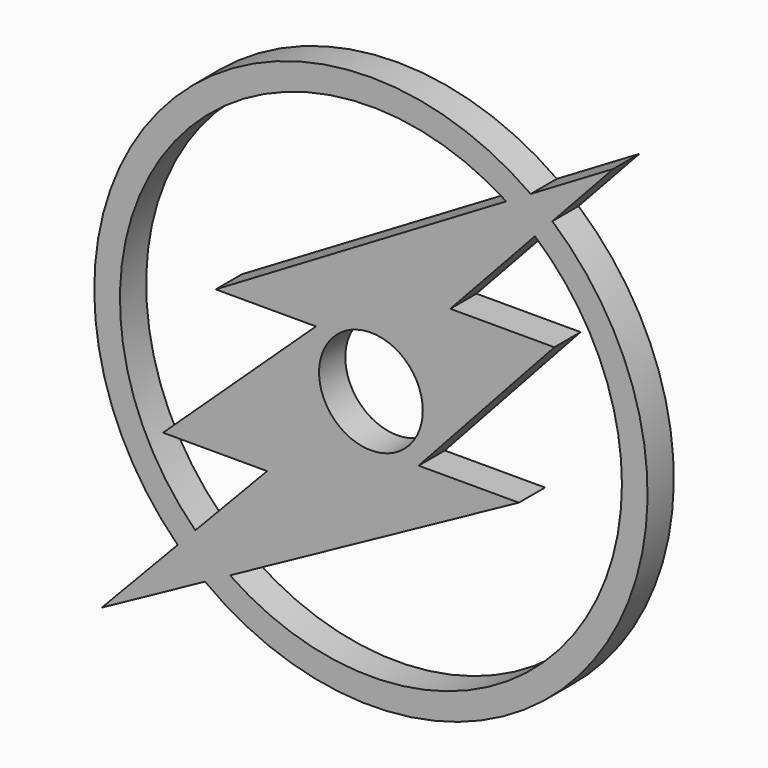
from build123d import *

# Parameters (mm, degrees)
F0_R     = 10.9728
F1_DEPTH = 6.9342


# Not quite as in the source:
# - a feature names something its author has since deleted; it is built from what else it names


with BuildPart() as f1:
    # F0 (on Front) → F1 (new body)
    with BuildSketch(Plane.XZ):
        with BuildLine():
            ThreePointArc((28.6439371533, 44.738406593), (31.7550616118, 42.5865732614), (34.7051660635, 40.2187967078))
            Line((34.7051660635, 40.2187967078), (38.3958422982, 44.2064153225))
            ThreePointArc((38.3958422982, 44.2064153225), (36.1509937048, 46.060324745), (33.8167671779, 47.8003568929))
            Line((33.8167671779, 47.8003568929), (28.6439371533, 44.738406593))
        make_face()
        with BuildLine():
            Line((38.3958422982, 44.2064153225), (34.7051660635, 40.2187967078))
            ThreePointArc((34.7051660635, 40.2187967078), (48.2991997583, 22.1175826623), (53.1225014483, 0))
            ThreePointArc((53.1225014483, 0), (24.8760182095, -46.9380855826), (-29.8247927528, -43.9600033823))
            Line((-29.8247927528, -43.9600033823), (-35.1168298869, -46.8535603786))
            ThreePointArc((-35.1168298869, -46.8535603786), (26.1940251259, -52.3671739658), (58.5529492123, 0))
            ThreePointArc((58.5529492123, 0), (53.2758747723, 24.2925714716), (38.3958422982, 44.2064153225))
        make_face()
        with BuildLine():
            ThreePointArc((33.8167671779, 47.8003568929), (36.1509937048, 46.060324745), (38.3958422982, 44.2064153225))
            Line((38.3958422982, 44.2064153225), (51.3007947444, 58.1496672696))
            Line((51.3007947444, 58.1496672696), (33.8167671779, 47.8003568929))
        make_face()
        with BuildLine():
            ThreePointArc((-37.1603482471, -37.9619372303), (-41.568846888, 33.0761413789), (28.6439371533, 44.738406593))
            Line((28.6439371533, 44.738406593), (33.8167671779, 47.8003568929))
            ThreePointArc((33.8167671779, 47.8003568929), (-44.9890332079, 37.475788884), (-40.9020715179, -41.898310312))
            Line((-40.9020715179, -41.898310312), (-37.1603482471, -37.9619372303))
        make_face()
        with BuildLine():
            Line((-35.1168298869, -46.8535603786), (-29.8247927528, -43.9600033823))
            ThreePointArc((-29.8247927528, -43.9600033823), (-33.6265739867, -41.1248547965), (-37.1603482471, -37.9619372303))
            Line((-37.1603482471, -37.9619372303), (-40.9020715179, -41.898310312))
            ThreePointArc((-40.9020715179, -41.898310312), (-38.090116415, -44.4701123559), (-35.1168298869, -46.8535603786))
        make_face()
        with BuildLine():
            Line((-56.9704473019, -58.8025860488), (-35.1168298869, -46.8535603786))
            ThreePointArc((-35.1168298869, -46.8535603786), (-38.090116415, -44.4701123559), (-40.9020715179, -41.898310312))
            Line((-40.9020715179, -41.898310312), (-56.9704473019, -58.8025860488))
        make_face()
        with BuildLine():
            Line((38.8165365087, 20.8673397533), (16.7947365087, 20.8673397533))
            Line((16.7947365087, 20.8673397533), (34.7051660635, 40.2187967078))
            ThreePointArc((34.7051660635, 40.2187967078), (31.7550616118, 42.5865732614), (28.6439371533, 44.738406593))
            Line((28.6439371533, 44.738406593), (-32.8515800228, 8.3374004968))
            Line((-32.8515800228, 8.3374004968), (-11.6390858311, 8.3374004968))
            Line((-11.6390858311, 8.3374004968), (-43.993112864, -21.982746443))
            Line((-43.993112864, -21.982746443), (-21.971312864, -21.982746443))
            Line((-21.971312864, -21.982746443), (-37.1603482471, -37.9619372303))
            ThreePointArc((-37.1603482471, -37.9619372303), (-33.6265739867, -41.1248547965), (-29.8247927528, -43.9600033823))
            Line((-29.8247927528, -43.9600033823), (31.308234758, -10.5339530787))
            Line((31.308234758, -10.5339530787), (10.099234758, -10.5339530787))
            Line((10.099234758, -10.5339530787), (38.8165365087, 20.8673397533))
        make_face()
        Circle(F0_R, mode=Mode.SUBTRACT)
    extrude(amount=F1_DEPTH)


solid = f1.part
